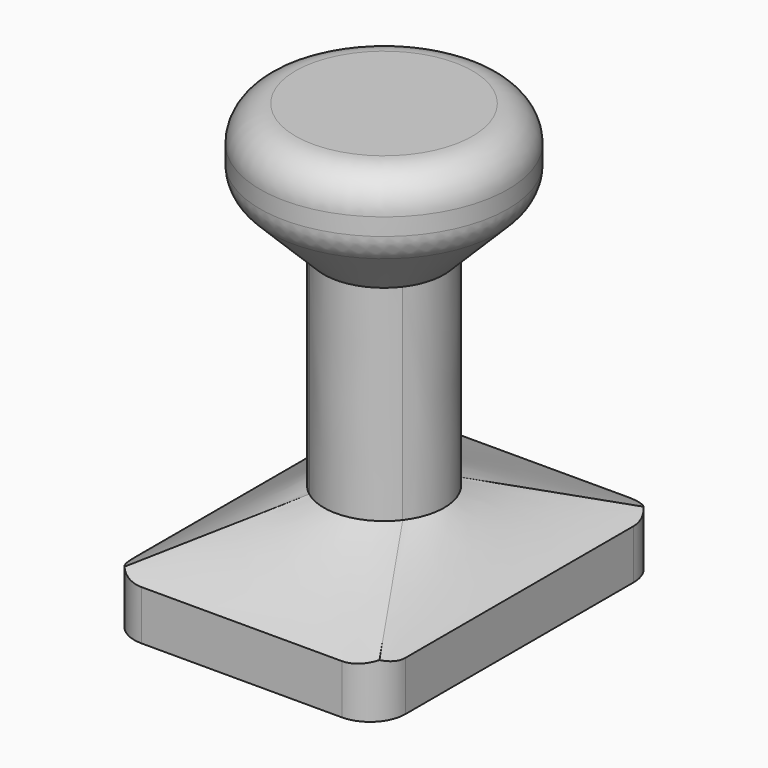
from build123d import *

# Parameters (mm, degrees)
F0_W      = 38.3
F0_H      = 50.3
F0_W_2    = 28.3
F0_H_2    = 40.3
F4_DEPTH  = 4
F5_DEPTH  = 3
F5_FACE_W = 38.3
F5_FACE_H = 50.3
F7_DEPTH  = 35
F9_DEPTH  = 8
F10_R     = 5
F11_R     = 5


# Not quite as in the source:
# - the arcs of a loft's sections are written as splines that run evenly, so that the points pair up as in the source's solid


with BuildPart() as f4:
    # F0 (on Top) → F4 (new body)
    with BuildSketch(Plane.XY):
        Rectangle(F0_W, F0_H)
        Rectangle(F0_W_2, F0_H_2, mode=Mode.SUBTRACT)
    extrude(amount=-F4_DEPTH)

    # F0 (on Top) → F5 (join)
    with BuildSketch(Plane.XY):
        Rectangle(F0_W, F0_H)
        Rectangle(F0_W_2, F0_H_2, mode=Mode.SUBTRACT)
        Rectangle(F0_W_2, F0_H_2)
    extrude(amount=F5_DEPTH)

    # F5_face (on face) → F6 section 0
    with BuildSketch(Plane.XY.offset(3)):
        Rectangle(F5_FACE_W, F5_FACE_H)
    # F2 (on offset) → F6 section 1
    with BuildSketch(Plane.XY.offset(10)):
        with BuildLine():
            add(Edge.make_bspline(
                [(5.1493417049, 6.762712474), (4.2641047121, 7.436759727), (3.2451924408, 7.934526467), (1.09359433, 8.5024723272), (-0.0382449475, 8.5724279849), (-2.2434058754, 8.2737605906), (-3.3158598892, 7.9052550514), (-5.2388678728, 6.785443806), (-6.0886652211, 6.0345786977), (-6.762712474, 5.1493417049)],
                knots=[0, 0, 0, 0, 0.25, 0.25, 0.5, 0.5, 0.75, 0.75, 1, 1, 1, 1], degree=3))
            add(Edge.make_bspline(
                [(-6.762712474, 5.1493417049), (-7.436759727, 4.2641047121), (-7.934526467, 3.2451924408), (-8.5024723272, 1.09359433), (-8.5724279849, -0.0382449475), (-8.2737605906, -2.2434058754), (-7.9052550514, -3.3158598892), (-6.785443806, -5.2388678728), (-6.0345786977, -6.0886652211), (-5.1493417049, -6.762712474)],
                knots=[0, 0, 0, 0, 0.25, 0.25, 0.5, 0.5, 0.75, 0.75, 1, 1, 1, 1], degree=3))
            add(Edge.make_bspline(
                [(-5.1493417049, -6.762712474), (-4.2641047121, -7.436759727), (-3.2451924408, -7.934526467), (-1.09359433, -8.5024723272), (0.0382449475, -8.5724279849), (2.2434058754, -8.2737605906), (3.3158598892, -7.9052550514), (5.2388678728, -6.785443806), (6.0886652211, -6.0345786977), (6.762712474, -5.1493417049)],
                knots=[0, 0, 0, 0, 0.25, 0.25, 0.5, 0.5, 0.75, 0.75, 1, 1, 1, 1], degree=3))
            add(Edge.make_bspline(
                [(6.762712474, -5.1493417049), (7.436759727, -4.2641047121), (7.934526467, -3.2451924408), (8.5024723272, -1.09359433), (8.5724279849, 0.0382449475), (8.2737605906, 2.2434058754), (7.9052550514, 3.3158598892), (6.785443806, 5.2388678728), (6.0345786977, 6.0886652211), (5.1493417049, 6.762712474)],
                knots=[0, 0, 0, 0, 0.25, 0.25, 0.5, 0.5, 0.75, 0.75, 1, 1, 1, 1], degree=3))
        make_face()
    loft(ruled=True)

    # F7 (add): a face of the model
    f7_faces = [f4.faces().sort_by_distance(p)[0] for p in [
        (0, 0, 10),
    ]]
    extrude(f7_faces, amount=F7_DEPTH)

    # F3 (on Front) → F8 (revolve)
    with BuildSketch(Plane.XZ):
        with BuildLine():
            Line((0, 30.5), (0, 65.5))
            ThreePointArc((0, 65.5), (-12.3743686708, 60.3743686708), (-17.5, 48))
            Line((-17.5, 48), (0, 30.5))
        make_face()
        with BuildLine():
            ThreePointArc((-17.5, 48), (-12.3743686708, 60.3743686708), (0, 65.5))
            Line((0, 65.5), (-17.5, 65.5))
            Line((-17.5, 65.5), (-17.5, 48))
        make_face()
    revolve(axis=Axis((0, 0, 48), (0, 0, -1)))

    # F9 (cut): a face of the model
    f9_faces = [f4.faces().sort_by_distance(p)[0] for p in [
        (0, 0, 65.5),
    ]]
    extrude(f9_faces, amount=-F9_DEPTH, mode=Mode.SUBTRACT)

    # F10
    f10_edges = [f4.edges().sort_by_distance(p)[0] for p in [
        (17.5, 0, 57.5),
        (17.5, 0, 48),
    ]]
    fillet(f10_edges, radius=F10_R)

    # F11
    f11_edges = [f4.edges().sort_by_distance(p)[0] for p in [
        (-19.15, -25.15, -0.5),
        (-19.15, 25.15, -0.5),
        (19.15, 25.15, -0.5),
        (19.15, -25.15, -0.5),
    ]]
    fillet(f11_edges, radius=F11_R)


solid = f4.part
